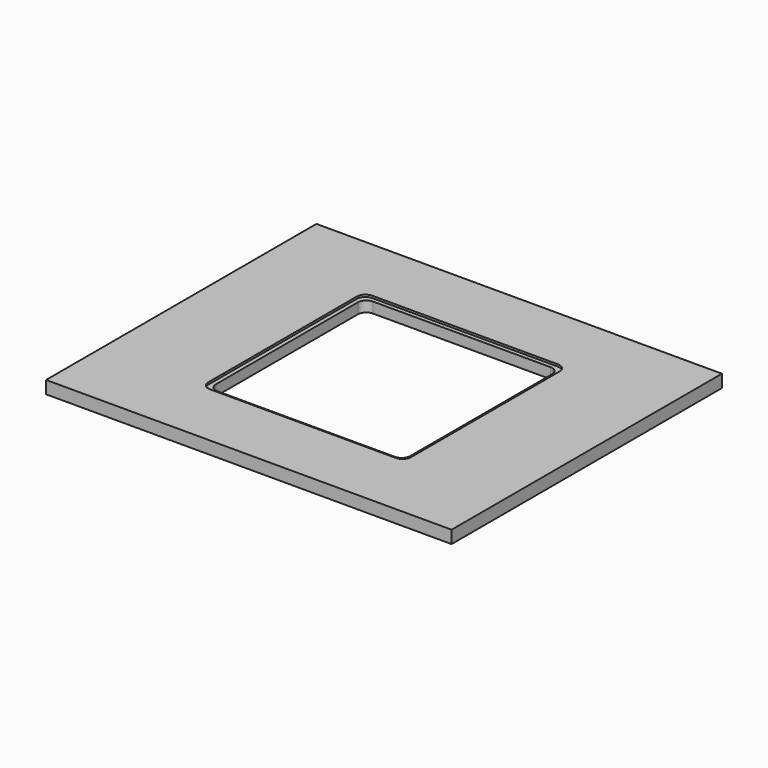
from build123d import *

# Parameters (mm, degrees)
F0_W     = 609.6
F0_H     = 508
F1_DEPTH = 19.05
F3_DEPTH = 3.175
F5_DEPTH = 19.05
F6_W     = 438.15
F6_H     = 19.05
F7_DEPTH = 6.35


# Not quite as in the source:
# - a length typed as a fraction of an inch, garbled in the dataset ("3 / 203.2 mm" for 3/8 in), is restored


with BuildPart() as f1:
    # F0 (on Top) → F1 (new body)
    with BuildSketch(Plane.XY):
        Rectangle(F0_W, F0_H)
    extrude(amount=F1_DEPTH)

    # F2 (on face) → F3 (cut)
    with BuildSketch(Plane.XY.offset(19.05)):
        with BuildLine():
            ThreePointArc((152.4, 139.7), (148.6802561211, 148.6802561211), (139.7, 152.4))
            Line((139.7, 152.4), (-139.7, 152.4))
            ThreePointArc((-139.7, 152.4), (-148.6802561211, 148.6802561211), (-152.4, 139.7))
            Line((-152.4, 139.7), (-152.4, -139.7))
            ThreePointArc((-152.4, -139.7), (-148.6802561211, -148.6802561211), (-139.7, -152.4))
            Line((-139.7, -152.4), (139.7, -152.4))
            ThreePointArc((139.7, -152.4), (148.6802561211, -148.6802561211), (152.4, -139.7))
            Line((152.4, -139.7), (152.4, 139.7))
        make_face()
    extrude(amount=-F3_DEPTH, mode=Mode.SUBTRACT)

    # F4 (on face) → F5 (cut)
    with BuildSketch(Plane.XY.offset(15.875)):
        with BuildLine():
            ThreePointArc((146.05, 133.35), (142.3302561211, 142.3302561211), (133.35, 146.05))
            Line((133.35, 146.05), (-133.35, 146.05))
            ThreePointArc((-133.35, 146.05), (-142.3302561211, 142.3302561211), (-146.05, 133.35))
            Line((-146.05, 133.35), (-146.05, -133.35))
            ThreePointArc((-146.05, -133.35), (-142.3302561211, -142.3302561211), (-133.35, -146.05))
            Line((-133.35, -146.05), (133.35, -146.05))
            ThreePointArc((133.35, -146.05), (142.3302561211, -142.3302561211), (146.05, -133.35))
            Line((146.05, -133.35), (146.05, 133.35))
        make_face()
    extrude(amount=-F5_DEPTH, mode=Mode.SUBTRACT)

    # F6 (on face) → F7 (cut)
    with BuildSketch(Plane(origin=(0, 0, 0), x_dir=(1, 0, 0), z_dir=(0, 0, -1))):
        Polygon((-219.075, 228.6), (-238.125, 228.6), (-238.125, -228.6), (-219.075, -228.6), (-219.075, -209.55), align=None)
        with Locations((0, -219.075)):
            Rectangle(F6_W, F6_H)
        Polygon((219.075, 228.6), (219.075, -209.55), (219.075, -228.6), (238.125, -228.6), (238.125, 228.6), align=None)
    extrude(amount=-F7_DEPTH, mode=Mode.SUBTRACT)


solid = f1.part
